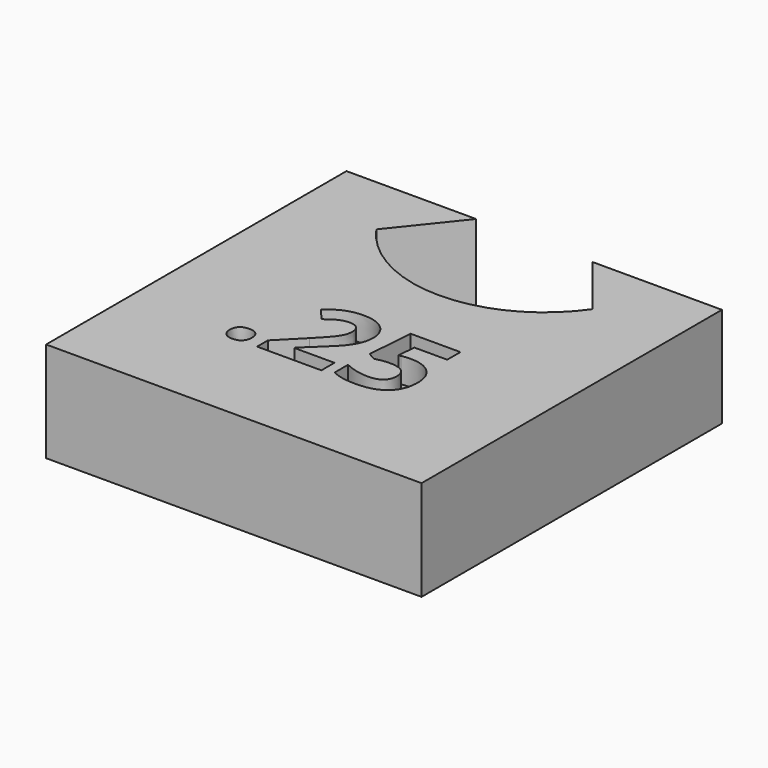
from build123d import *

# Parameters (mm, degrees)
F1_DEPTH     = 4
F2_TEXT_SIZE = 5.1441598549
F3_DEPTH     = 1


# Not quite as in the source:
# - Text() gives the source's letters only with a copy of the font that has no kerning and outlines rounded to 1/6400 em; it was checked with that copy


with BuildPart() as f1:
    # F0 (on Top) → F1 (new body)
    with BuildSketch(Plane.XY):
        with BuildLine():
            Line((7.5, -7.5), (7.5, 7.5))
            Line((7.5, 7.5), (2.3201562119, 7.5))
            Line((2.3201562119, 7.5), (4.3138768579, 5.0078491925))
            ThreePointArc((4.3138768579, 5.0078491925), (2.4345131198, 3.3485866804), (0, 2.75))
            ThreePointArc((0, 2.75), (-2.4345131198, 3.3485866804), (-4.3138768579, 5.0078491925))
            Line((-4.3138768579, 5.0078491925), (-2.3201562119, 7.5))
            Line((-2.3201562119, 7.5), (-7.5, 7.5))
            Line((-7.5, 7.5), (-7.5, -7.5))
            Line((-7.5, -7.5), (7.5, -7.5))
        make_face()
    extrude(amount=F1_DEPTH)

    # F2 (on face) → F3 (cut)
    with BuildSketch(Plane.XY.offset(4)):
        with Locations((-3.9421525151, -3.5)):
            Text('.25', F2_TEXT_SIZE, font='Open Sans', font_style=FontStyle.BOLD, text_align=(TextAlign.LEFT, TextAlign.BOTTOM))
    extrude(amount=-F3_DEPTH, mode=Mode.SUBTRACT)


solid = f1.part
